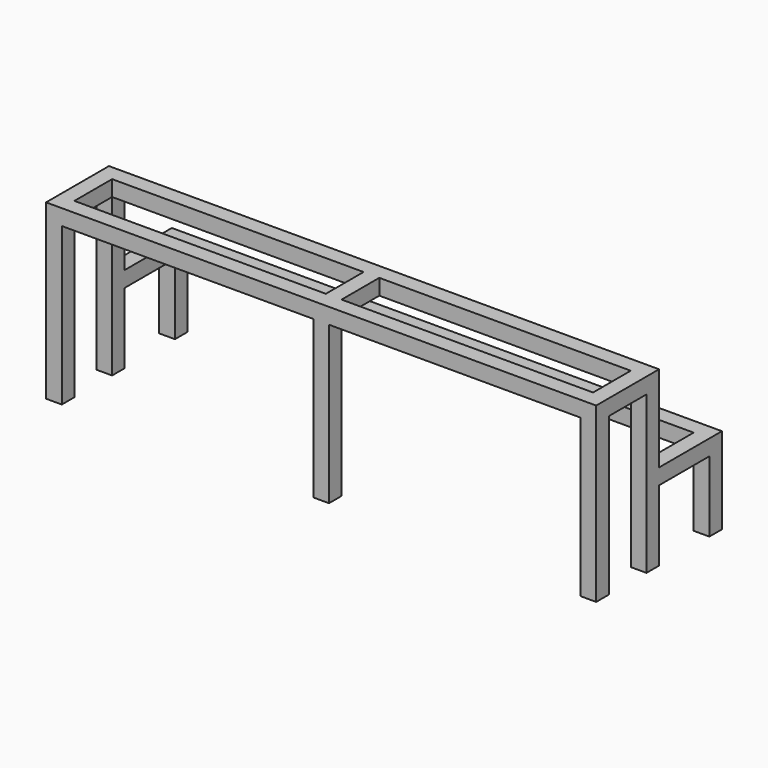
from build123d import *

# Parameters (mm, degrees)
F0_W      = 1400
F0_H      = 200
F0_W_2    = 40
F0_H_2    = 120
F1_DEPTH  = 40
F2_W      = 40
F2_H      = 40
F3_DEPTH  = 400
F4_W      = 40
F4_H      = 40
F5_DEPTH  = 200
F7_W      = 40
F7_H      = 40
F6_W      = 40
F6_H      = 40
F8_DEPTH  = 180
F9_W      = 40
F9_H      = 40
F10_DEPTH = 1320


# Not quite as in the source:
# - a feature names something its author has since deleted; it is built from what else it names


with BuildPart() as f1:
    # F0 (on Top) → F1 (new body)
    with BuildSketch(Plane.XY):
        Rectangle(F0_W, F0_H)
        Polygon((20, 60), (660, 60), (660, -60), (20, -60), (-20, -60), (-660, -60), (-660, 60), (-20, 60), align=None, mode=Mode.SUBTRACT)
        Rectangle(F0_W_2, F0_H_2)
    extrude(amount=F1_DEPTH)

    # F2 (on face) → F3 (join)
    with BuildSketch(Plane(origin=(0, 0, 0), x_dir=(1, 0, 0), z_dir=(0, 0, -1))):
        with Locations((-680, 80)):
            Rectangle(F2_W, F2_H)
        with Locations((-680, -80)):
            Rectangle(F2_W, F2_H)
        with Locations((680, 80)):
            Rectangle(F2_W, F2_H)
        with Locations((680, -80)):
            Rectangle(F2_W, F2_H)
        with Locations((0, 80)):
            Rectangle(F2_W, F2_H)
    extrude(amount=F3_DEPTH)

    # F4 (on face) → F5 (join)
    with BuildSketch(Plane(origin=(0, 100, 0), x_dir=(-1, 0, 0), z_dir=(0, 1, 0))):
        with Locations((-680, -200)):
            Rectangle(F4_W, F4_H)
        with Locations((680, -200)):
            Rectangle(F4_W, F4_H)
    extrude(amount=F5_DEPTH)

    # F7 (on face) + F6 (on face) → F8 (join)
    with BuildSketch(Plane(origin=(0, 0, -220), x_dir=(1, 0, 0), z_dir=(0, 0, -1))):
        with Locations((680, -280)):
            Rectangle(F7_W, F7_H)
    with BuildSketch(Plane(origin=(0, 0, -220), x_dir=(1, 0, 0), z_dir=(0, 0, -1))):
        with Locations((-680, -280)):
            Rectangle(F6_W, F6_H)
    extrude(amount=F8_DEPTH)

    # F9 (on face) → F10 (join, through all)
    with BuildSketch(Plane(origin=(660, 0, 0), x_dir=(0, -1, 0), z_dir=(-1, 0, 0))):
        with Locations((-280, -200)):
            Rectangle(F9_W, F9_H)
    extrude(amount=F10_DEPTH)


solid = f1.part
